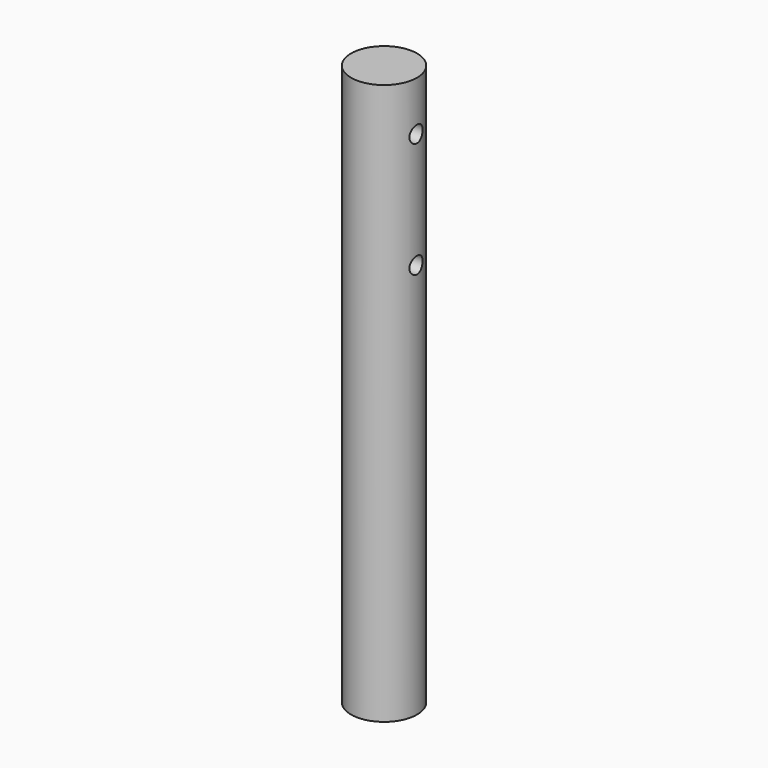
from build123d import *

# Parameters (mm, degrees)
F0_R     = 12.7
F1_DEPTH = 215.9
F2_R     = 3.175
F3_DEPTH = 12.7


with BuildPart() as f1:
    # F0 (on Top) → F1 (new body)
    with BuildSketch(Plane.XY):
        Circle(F0_R)
    extrude(amount=-F1_DEPTH)

    # F2 (on Right) → F3 (cut, symmetric)
    with BuildSketch(Plane.YZ):
        with Locations((0, -19.05)):
            Circle(F2_R)
        with Locations((0, -63.5)):
            Circle(F2_R)
    extrude(amount=F3_DEPTH, both=True, mode=Mode.SUBTRACT)


solid = f1.part
